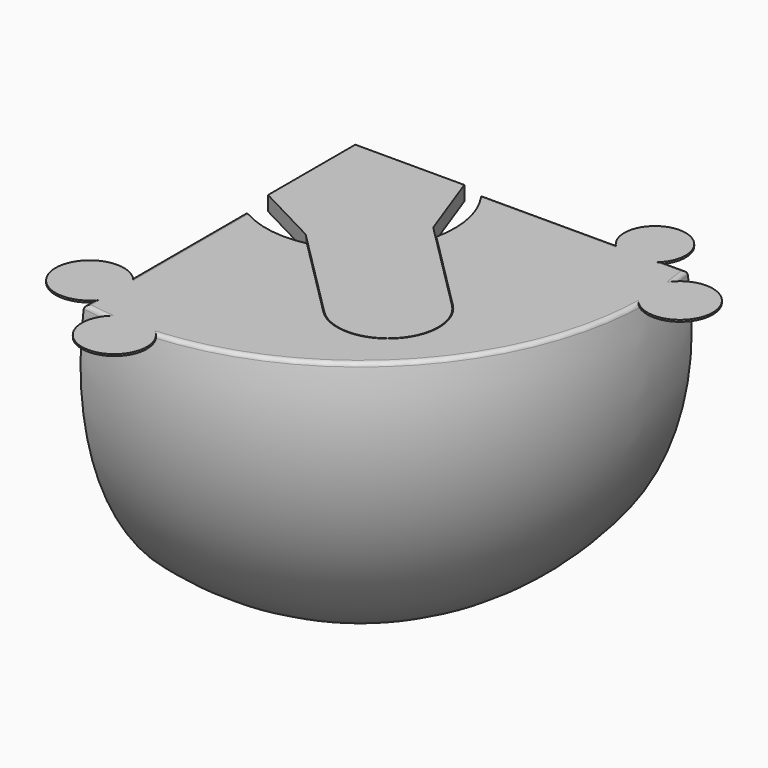
from build123d import *

# Parameters (mm, degrees)
F3_DEPTH  = 127
F5_DEPTH  = 254
F8_SIZE   = 7.62
F10_DEPTH = 10.16
F11_R     = 5.07999
F12_R     = 1.524
F14_DEPTH = 5.08
F15_R     = 11.4157397534
F15_R_2   = 10.7235303576
F15_R_3   = 11.3685520534
F15_R_4   = 11.9107845334
F16_DEPTH = 0.635


# Not quite as in the source:
# - a fillet or chamfer is up to 0.001 mm smaller than in the source, because OpenCascade refuses the exact size


with BuildPart() as f1:
    # F0 (on Front) → F1 (revolve)
    with BuildSketch(Plane.XZ):
        with BuildLine():
            ThreePointArc((17.78, -101.6), (119.38, 0), (17.78, 101.6))
            Line((17.78, 101.6), (17.78, -101.6))
        make_face()
    revolve(axis=Axis((17.78, 0, 0), (0, 0, -1)))

    # F2 (on Front) → F3 (cut, symmetric)
    with BuildSketch(Plane.XZ):
        with BuildLine():
            Line((0, -149.136774605), (0, 17.78))
            Line((0, 17.78), (166.8577827513, 17.78))
            ThreePointArc((166.8577827513, 17.78), (-88.4894929474, 106.1792374941), (0, -149.136774605))
        make_face()
    extrude(amount=F3_DEPTH, both=True, mode=Mode.SUBTRACT)

    # F4 (on Right) → F5 (cut, symmetric)
    with BuildSketch(Plane.YZ):
        Polygon((156.3395333682, 38.1), (20.32, 38.1), (20.32, 17.78), (20.32, -154.5686624048), (156.3395333682, -154.5686624048), align=None)
    extrude(amount=F5_DEPTH, both=True, mode=Mode.SUBTRACT)

    # F6 (on Front) → F7 (revolve, cut)
    with BuildSketch(Plane.XZ):
        Polygon((50.8, 17.78), (17.78, 17.78), (17.78, -96.52), (85.5823882628, -68.6945889125), (109.22, -30.9004336539), (109.22, 13.97), (50.8, 13.97), align=None)
    revolve(axis=Axis((17.78, 0, 0), (0, 0, -1)), mode=Mode.SUBTRACT)

    # F8
    f8_edges = [f1.edges().sort_by_distance(p)[0] for p in [
        (0, 20.32, -91.692902),
    ]]
    chamfer(f8_edges, length=F8_SIZE)

    # F9 (on face) → F10 (cut)
    with BuildSketch(Plane.XY.offset(17.78)):
        with BuildLine():
            ThreePointArc((30.3523585695, 12.5723585695), (5.2076414305, 12.5723585695), (5.2076414305, -12.5723585695))
            Line((5.2076414305, -12.5723585695), (53.7010244843, -61.0657416233))
            ThreePointArc((53.7010244843, -61.0657416233), (78.8457416233, -61.0657416233), (78.8457416233, -35.9210244843))
            Line((78.8457416233, -35.9210244843), (30.3523585695, 12.5723585695))
        make_face()
    extrude(amount=-F10_DEPTH, mode=Mode.SUBTRACT)

    # F11 (radius 5.08 in the source; OpenCascade refuses exactly that, so slightly less here)
    f11_edges = [f1.edges().sort_by_distance(p)[0] for p in [
        (83.349501, -63.733148, 13.97),
    ]]
    fillet(f11_edges, radius=F11_R)

    # F12
    f12_edges = [f1.edges().sort_by_distance(p)[0] for p in [
        (0, -63.131822, 17.78),
        (79.766909, 20.32, 17.78),
        (81.919925, -76.762632, 17.78),
        (117.289389, 10.213375, 17.78),
    ]]
    fillet(f12_edges, radius=F12_R)

    # F15 (on face) → F16 (join)
    with BuildSketch(Plane.XY.offset(17.78)):
        with Locations((125.4964470863, 5.0220037811)):
            Circle(F15_R)
        with Locations((99.333524704, 26.7573595047)):
            Circle(F15_R_2)
        with Locations((17.6246780902, -107.277341187)):
            Circle(F15_R_3)
        with Locations((-7.7332337387, -86.3469913602)):
            Circle(F15_R_4)
    extrude(amount=-F16_DEPTH)


with BuildPart() as f14:
    # F13 (on face) → F14 (new body)
    with BuildSketch(Plane.XY.offset(17.78)):
        with BuildLine():
            Line((21.2537209734, -28.2592278675), (5.3872465529, -12.3927534471))
            ThreePointArc((5.3872465529, -12.3927534471), (5.3872465529, 12.3927534471), (30.1727534471, 12.3927534471))
            Line((30.1727534471, 12.3927534471), (45.9027885404, -3.3372816463))
            Line((45.9027885404, -3.3372816463), (36.83, 21.59))
            Line((36.83, 21.59), (-1.27, 21.59))
            Line((-1.27, 21.59), (-1.27, -16.51))
            Line((-1.27, -16.51), (21.2537209734, -28.2592278675))
        make_face()
        with BuildLine():
            ThreePointArc((30.1727534471, 12.3927534471), (5.3872465529, 12.3927534471), (5.3872465529, -12.3927534471))
            Line((5.3872465529, -12.3927534471), (21.2537209734, -28.2592278675))
            Line((21.2537209734, -28.2592278675), (53.8806296067, -60.8861365008))
            ThreePointArc((53.8806296067, -60.8861365008), (78.6661365008, -60.8861365008), (78.6661365008, -36.1006296067))
            Line((78.6661365008, -36.1006296067), (45.9027885404, -3.3372816463))
            Line((45.9027885404, -3.3372816463), (30.1727534471, 12.3927534471))
        make_face()
    extrude(amount=-F14_DEPTH)


solid = Compound([f1.part, f14.part])
